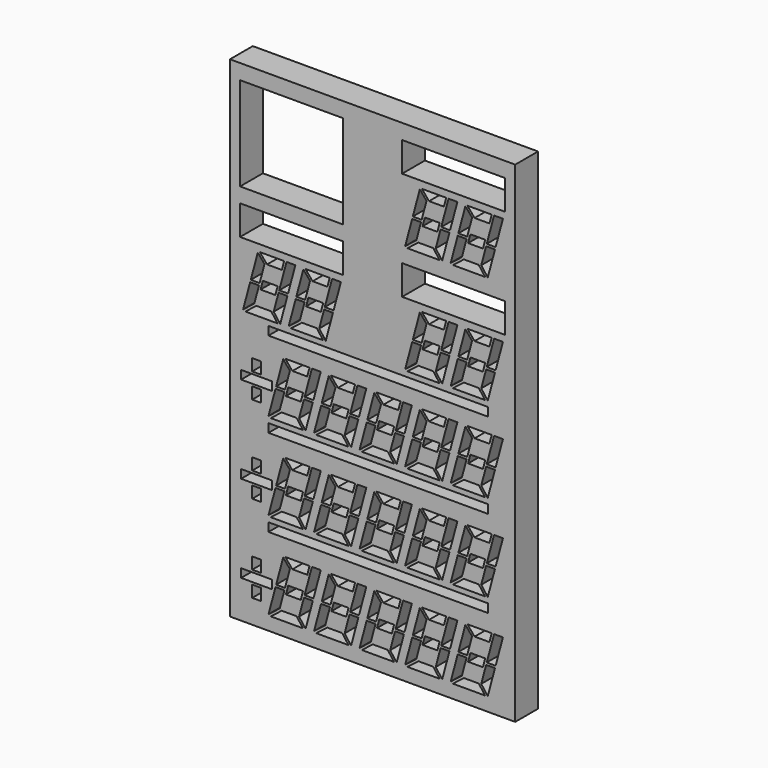
from build123d import *

# Parameters (mm, degrees)
F0_W     = 63.5
F0_H     = 109.22
F1_DEPTH = 6.35
F2_W     = 48.8092640617
F2_H     = 1.905
F2_W_2   = 1.905
F2_H_2   = 2.6035
F2_W_3   = 22.86
F2_H_3   = 6.604
F2_H_4   = 20.828
F3_DEPTH = 6.351


# Not quite as in the source:
# - a feature of the source that left no trace in its solid (it failed there, or was rolled back) is left out


with BuildPart() as f1:
    # F0 (on Front) → F1 (new body)
    with BuildSketch(Plane.XZ):
        Rectangle(F0_W, F0_H)
    extrude(amount=F1_DEPTH)

    # F2 (on face) → F3 (cut, through all)
    with BuildSketch(Plane.XZ.offset(6.35)):
        Polygon((26.5213785767, -38.9255), (21.1104505677, -38.9255), (22.7089353651, -40.8305), (26.0109353651, -40.8305), align=None)
        Polygon((29.0195, -38.9255), (27.0472988763, -38.9255), (25.4138805993, -45.0215), (27.3860817229, -45.0215), align=None)
        Polygon((27.2499635332, -45.5295), (25.2777624095, -45.5295), (24.1836844814, -49.6126544151), (25.6385600829, -51.5433395481), align=None)
        Polygon((22.1498008505, -40.9544571376), (20.6549496749, -39.1729628786), (19.0878388763, -45.0215), (21.06004, -45.0215), align=None)
        Polygon((17.888578235, -51.6255), (25.0643875098, -51.6255), (23.6288670444, -49.7205), (20.3268670444, -49.7205), align=None)
        Polygon((19.8801693423, -49.4248372408), (20.9239218102, -45.5295), (18.9517206865, -45.5295), (17.3857808211, -51.3736671393), align=None)
        Polygon((25.0751228105, -44.323), (21.7731228105, -44.323), (21.2626795989, -46.228), (24.5646795989, -46.228), align=None)
        Polygon((21.7731228105, -24.892), (21.2626795989, -26.797), (24.5646795989, -26.797), (25.0751228105, -24.892), align=None)
        Polygon((20.9239218102, -26.0985), (18.9517206865, -26.0985), (17.3857808211, -31.9426671393), (19.8801693423, -29.9938372408), align=None)
        Polygon((21.06004, -25.5905), (22.1498008505, -21.5234571376), (20.6549496749, -19.7419628786), (19.0878388763, -25.5905), align=None)
        Polygon((27.3860817229, -25.5905), (29.0195, -19.4945), (27.0472988763, -19.4945), (25.4138805993, -25.5905), align=None)
        Polygon((22.7089353651, -21.3995), (26.0109353651, -21.3995), (26.5213785767, -19.4945), (21.1104505677, -19.4945), align=None)
        Polygon((17.888578235, -32.1945), (25.0643875098, -32.1945), (23.6288670444, -30.2895), (20.3268670444, -30.2895), align=None)
        Polygon((27.2499635332, -26.0985), (25.2777624095, -26.0985), (24.1836844814, -30.1816544151), (25.6385600829, -32.1123395481), align=None)
        Polygon((21.7731228105, -5.461), (21.2626795989, -7.366), (24.5646795989, -7.366), (25.0751228105, -5.461), align=None)
        Polygon((20.9239218102, -6.6675), (18.9517206865, -6.6675), (17.3857808211, -12.5116671393), (19.8801693423, -10.5628372408), align=None)
        Polygon((21.06004, -6.1595), (22.1498008505, -2.0924571376), (20.6549496749, -0.3109628786), (19.0878388763, -6.1595), align=None)
        Polygon((27.3860817229, -6.1595), (29.0195, -0.0635), (27.0472988763, -0.0635), (25.4138805993, -6.1595), align=None)
        Polygon((22.7089353651, -1.9685), (26.0109353651, -1.9685), (26.5213785767, -0.0635), (21.1104505677, -0.0635), align=None)
        Polygon((17.888578235, -12.7635), (25.0643875098, -12.7635), (23.6288670444, -10.8585), (20.3268670444, -10.8585), align=None)
        Polygon((27.2499635332, -6.6675), (25.2777624095, -6.6675), (24.1836844814, -10.7506544151), (25.6385600829, -12.6813395481), align=None)
        Polygon((11.6340016105, -44.323), (11.1235583989, -46.228), (14.4255583989, -46.228), (14.9360016105, -44.323), align=None)
        Polygon((10.7848006102, -45.5295), (8.8125994865, -45.5295), (7.2466596211, -51.3736671393), (9.7410481423, -49.4248372408), align=None)
        Polygon((10.9209188, -45.0215), (12.0106796505, -40.9544571376), (10.5158284749, -39.1729628786), (8.9487176763, -45.0215), align=None)
        Polygon((17.2469605229, -45.0215), (18.8803788, -38.9255), (16.9081776763, -38.9255), (15.2747593993, -45.0215), align=None)
        Polygon((12.5698141651, -40.8305), (15.8718141651, -40.8305), (16.3822573767, -38.9255), (10.9713293677, -38.9255), align=None)
        Polygon((7.749457035, -51.6255), (14.9252663098, -51.6255), (13.4897458444, -49.7205), (10.1877458444, -49.7205), align=None)
        Polygon((17.1108423332, -45.5295), (15.1386412095, -45.5295), (14.0445632814, -49.6126544151), (15.4994388829, -51.5433395481), align=None)
        Polygon((11.6340016105, -24.892), (11.1235583989, -26.797), (14.4255583989, -26.797), (14.9360016105, -24.892), align=None)
        Polygon((10.7848006102, -26.0985), (8.8125994865, -26.0985), (7.2466596211, -31.9426671393), (9.7410481423, -29.9938372408), align=None)
        Polygon((10.9209188, -25.5905), (12.0106796505, -21.5234571376), (10.5158284749, -19.7419628786), (8.9487176763, -25.5905), align=None)
        Polygon((17.2469605229, -25.5905), (18.8803788, -19.4945), (16.9081776763, -19.4945), (15.2747593993, -25.5905), align=None)
        Polygon((12.5698141651, -21.3995), (15.8718141651, -21.3995), (16.3822573767, -19.4945), (10.9713293677, -19.4945), align=None)
        Polygon((7.749457035, -32.1945), (14.9252663098, -32.1945), (13.4897458444, -30.2895), (10.1877458444, -30.2895), align=None)
        Polygon((17.1108423332, -26.0985), (15.1386412095, -26.0985), (14.0445632814, -30.1816544151), (15.4994388829, -32.1123395481), align=None)
        Polygon((11.6340016105, -5.461), (11.1235583989, -7.366), (14.4255583989, -7.366), (14.9360016105, -5.461), align=None)
        Polygon((10.7848006102, -6.6675), (8.8125994865, -6.6675), (7.2466596211, -12.5116671393), (9.7410481423, -10.5628372408), align=None)
        Polygon((10.9209188, -6.1595), (12.0106796505, -2.0924571376), (10.5158284749, -0.3109628786), (8.9487176763, -6.1595), align=None)
        Polygon((17.2469605229, -6.1595), (18.8803788, -0.0635), (16.9081776763, -0.0635), (15.2747593993, -6.1595), align=None)
        Polygon((12.5698141651, -1.9685), (15.8718141651, -1.9685), (16.3822573767, -0.0635), (10.9713293677, -0.0635), align=None)
        Polygon((7.749457035, -12.7635), (14.9252663098, -12.7635), (13.4897458444, -10.8585), (10.1877458444, -10.8585), align=None)
        Polygon((17.1108423332, -6.6675), (15.1386412095, -6.6675), (14.0445632814, -10.7506544151), (15.4994388829, -12.6813395481), align=None)
        Polygon((1.4948804105, -44.323), (0.9844371989, -46.228), (4.2864371989, -46.228), (4.7968804105, -44.323), align=None)
        Polygon((0.6456794102, -45.5295), (-1.3265217135, -45.5295), (-2.8924615789, -51.3736671393), (-0.3980730577, -49.4248372408), align=None)
        Polygon((0.7817976, -45.0215), (1.8715584505, -40.9544571376), (0.3767072749, -39.1729628786), (-1.1904035237, -45.0215), align=None)
        Polygon((7.1078393229, -45.0215), (8.7412576, -38.9255), (6.7690564763, -38.9255), (5.1356381993, -45.0215), align=None)
        Polygon((2.4306929651, -40.8305), (5.7326929651, -40.8305), (6.2431361767, -38.9255), (0.8322081677, -38.9255), align=None)
        Polygon((-2.389664165, -51.6255), (4.7861451098, -51.6255), (3.3506246444, -49.7205), (0.0486246444, -49.7205), align=None)
        Polygon((6.9717211332, -45.5295), (4.9995200095, -45.5295), (3.9054420814, -49.6126544151), (5.3603176829, -51.5433395481), align=None)
        Polygon((1.4948804105, -24.892), (0.9844371989, -26.797), (4.2864371989, -26.797), (4.7968804105, -24.892), align=None)
        Polygon((0.6456794102, -26.0985), (-1.3265217135, -26.0985), (-2.8924615789, -31.9426671393), (-0.3980730577, -29.9938372408), align=None)
        Polygon((0.7817976, -25.5905), (1.8715584505, -21.5234571376), (0.3767072749, -19.7419628786), (-1.1904035237, -25.5905), align=None)
        Polygon((7.1078393229, -25.5905), (8.7412576, -19.4945), (6.7690564763, -19.4945), (5.1356381993, -25.5905), align=None)
        Polygon((2.4306929651, -21.3995), (5.7326929651, -21.3995), (6.2431361767, -19.4945), (0.8322081677, -19.4945), align=None)
        Polygon((-2.389664165, -32.1945), (4.7861451098, -32.1945), (3.3506246444, -30.2895), (0.0486246444, -30.2895), align=None)
        Polygon((6.9717211332, -26.0985), (4.9995200095, -26.0985), (3.9054420814, -30.1816544151), (5.3603176829, -32.1123395481), align=None)
        Polygon((1.4948804105, -5.461), (0.9844371989, -7.366), (4.2864371989, -7.366), (4.7968804105, -5.461), align=None)
        Polygon((0.6456794102, -6.6675), (-1.3265217135, -6.6675), (-2.8924615789, -12.5116671393), (-0.3980730577, -10.5628372408), align=None)
        Polygon((0.7817976, -6.1595), (1.8715584505, -2.0924571376), (0.3767072749, -0.3109628786), (-1.1904035237, -6.1595), align=None)
        Polygon((7.1078393229, -6.1595), (8.7412576, -0.0635), (6.7690564763, -0.0635), (5.1356381993, -6.1595), align=None)
        Polygon((2.4306929651, -1.9685), (5.7326929651, -1.9685), (6.2431361767, -0.0635), (0.8322081677, -0.0635), align=None)
        Polygon((-2.389664165, -12.7635), (4.7861451098, -12.7635), (3.3506246444, -10.8585), (0.0486246444, -10.8585), align=None)
        Polygon((6.9717211332, -6.6675), (4.9995200095, -6.6675), (3.9054420814, -10.7506544151), (5.3603176829, -12.6813395481), align=None)
        Polygon((-8.6442407895, -44.323), (-9.1546840011, -46.228), (-5.8526840011, -46.228), (-5.3422407895, -44.323), align=None)
        Polygon((-9.4934417898, -45.5295), (-11.4656429135, -45.5295), (-13.0315827789, -51.3736671393), (-10.5371942577, -49.4248372408), align=None)
        Polygon((-9.3573236, -45.0215), (-8.2675627495, -40.9544571376), (-9.7624139251, -39.1729628786), (-11.3295247237, -45.0215), align=None)
        Polygon((-3.0312818771, -45.0215), (-1.3978636, -38.9255), (-3.3700647237, -38.9255), (-5.0034830007, -45.0215), align=None)
        Polygon((-7.7084282349, -40.8305), (-4.4064282349, -40.8305), (-3.8959850233, -38.9255), (-9.3069130323, -38.9255), align=None)
        Polygon((-12.528785365, -51.6255), (-5.3529760902, -51.6255), (-6.7884965556, -49.7205), (-10.0904965556, -49.7205), align=None)
        Polygon((-3.1674000668, -45.5295), (-5.1396011905, -45.5295), (-6.2336791186, -49.6126544151), (-4.7788035171, -51.5433395481), align=None)
        Polygon((-8.6442407895, -24.892), (-9.1546840011, -26.797), (-5.8526840011, -26.797), (-5.3422407895, -24.892), align=None)
        Polygon((-9.4934417898, -26.0985), (-11.4656429135, -26.0985), (-13.0315827789, -31.9426671393), (-10.5371942577, -29.9938372408), align=None)
        Polygon((-9.3573236, -25.5905), (-8.2675627495, -21.5234571376), (-9.7624139251, -19.7419628786), (-11.3295247237, -25.5905), align=None)
        Polygon((-3.0312818771, -25.5905), (-1.3978636, -19.4945), (-3.3700647237, -19.4945), (-5.0034830007, -25.5905), align=None)
        Polygon((-7.7084282349, -21.3995), (-4.4064282349, -21.3995), (-3.8959850233, -19.4945), (-9.3069130323, -19.4945), align=None)
        Polygon((-12.528785365, -32.1945), (-5.3529760902, -32.1945), (-6.7884965556, -30.2895), (-10.0904965556, -30.2895), align=None)
        Polygon((-3.1674000668, -26.0985), (-5.1396011905, -26.0985), (-6.2336791186, -30.1816544151), (-4.7788035171, -32.1123395481), align=None)
        Polygon((-8.6442407895, -5.461), (-9.1546840011, -7.366), (-5.8526840011, -7.366), (-5.3422407895, -5.461), align=None)
        Polygon((-9.4934417898, -6.6675), (-11.4656429135, -6.6675), (-13.0315827789, -12.5116671393), (-10.5371942577, -10.5628372408), align=None)
        Polygon((-9.3573236, -6.1595), (-8.2675627495, -2.0924571376), (-9.7624139251, -0.3109628786), (-11.3295247237, -6.1595), align=None)
        Polygon((-3.0312818771, -6.1595), (-1.3978636, -0.0635), (-3.3700647237, -0.0635), (-5.0034830007, -6.1595), align=None)
        Polygon((-7.7084282349, -1.9685), (-4.4064282349, -1.9685), (-3.8959850233, -0.0635), (-9.3069130323, -0.0635), align=None)
        Polygon((-12.528785365, -12.7635), (-5.3529760902, -12.7635), (-6.7884965556, -10.8585), (-10.0904965556, -10.8585), align=None)
        Polygon((-3.1674000668, -6.6675), (-5.1396011905, -6.6675), (-6.2336791186, -10.7506544151), (-4.7788035171, -12.6813395481), align=None)
        Polygon((-19.0385835953, -45.2755), (-19.2938052011, -46.228), (-15.9918052011, -46.228), (-15.4813619895, -44.323), (-18.7833619895, -44.323), align=None)
        Polygon((-19.6325629898, -45.5295), (-21.6047641135, -45.5295), (-23.1707039789, -51.3736671393), (-20.6763154577, -49.4248372408), align=None)
        Polygon((-19.4964448, -45.0215), (-18.4066839495, -40.9544571376), (-19.9015351251, -39.1729628786), (-21.4686459237, -45.0215), align=None)
        Polygon((-13.1704030771, -45.0215), (-11.5369848, -38.9255), (-13.5091859237, -38.9255), (-15.1426042007, -45.0215), align=None)
        Polygon((-17.8475494349, -40.8305), (-14.5455494349, -40.8305), (-14.0351062233, -38.9255), (-19.4460342323, -38.9255), align=None)
        Polygon((-22.667906565, -51.6255), (-15.4920972902, -51.6255), (-16.9276177556, -49.7205), (-20.2296177556, -49.7205), align=None)
        Polygon((-13.3065212668, -45.5295), (-15.2787223905, -45.5295), (-16.3728003186, -49.6126544151), (-14.9179247171, -51.5433395481), align=None)
        Polygon((-18.7833619895, -24.892), (-19.2938052011, -26.797), (-15.9918052011, -26.797), (-15.4813619895, -24.892), align=None)
        Polygon((-19.6325629898, -26.0985), (-21.6047641135, -26.0985), (-23.1707039789, -31.9426671393), (-20.6763154577, -29.9938372408), align=None)
        Polygon((-19.4964448, -25.5905), (-18.4066839495, -21.5234571376), (-19.9015351251, -19.7419628786), (-21.4686459237, -25.5905), align=None)
        Polygon((-13.1704030771, -25.5905), (-11.5369848, -19.4945), (-13.5091859237, -19.4945), (-15.1426042007, -25.5905), align=None)
        Polygon((-17.8475494349, -21.3995), (-14.5455494349, -21.3995), (-14.0351062233, -19.4945), (-19.4460342323, -19.4945), align=None)
        Polygon((-22.667906565, -32.1945), (-15.4920972902, -32.1945), (-16.9276177556, -30.2895), (-20.2296177556, -30.2895), align=None)
        Polygon((-13.3065212668, -26.0985), (-15.2787223905, -26.0985), (-16.3728003186, -30.1816544151), (-14.9179247171, -32.1123395481), align=None)
        Polygon((-18.7833619895, -5.461), (-19.2938052011, -7.366), (-15.9918052011, -7.366), (-15.4813619895, -5.461), align=None)
        Polygon((-19.6325629898, -6.6675), (-21.6047641135, -6.6675), (-23.1707039789, -12.5116671393), (-20.6763154577, -10.5628372408), align=None)
        Polygon((-19.4964448, -6.1595), (-18.4066839495, -2.0924571376), (-19.9015351251, -0.3109628786), (-21.4686459237, -6.1595), align=None)
        Polygon((-13.1704030771, -6.1595), (-11.5369848, -0.0635), (-13.5091859237, -0.0635), (-15.1426042007, -6.1595), align=None)
        Polygon((-17.8475494349, -1.9685), (-14.5455494349, -1.9685), (-14.0351062233, -0.0635), (-19.4460342323, -0.0635), align=None)
        Polygon((-22.667906565, -12.7635), (-15.4920972902, -12.7635), (-16.9276177556, -10.8585), (-20.2296177556, -10.8585), align=None)
        Polygon((-13.3065212668, -6.6675), (-15.2787223905, -6.6675), (-16.3728003186, -10.7506544151), (-14.9179247171, -12.6813395481), align=None)
        Polygon((22.7089353651, 17.0815), (26.0109353651, 17.0815), (26.5213785767, 18.9865), (21.1104505677, 18.9865), align=None)
        Polygon((21.7731228105, 13.589), (21.2626795989, 11.684), (24.5646795989, 11.684), (25.0751228105, 13.589), align=None)
        Polygon((12.5698141651, 17.0815), (15.8718141651, 17.0815), (16.3822573767, 18.9865), (10.9713293677, 18.9865), align=None)
        Polygon((29.0195, 18.9865), (27.0472988763, 18.9865), (25.4138805993, 12.8905), (27.3860817229, 12.8905), align=None)
        Polygon((18.9517206865, 12.3825), (17.3857808211, 6.5383328607), (19.8801693423, 8.4871627592), (20.9239218102, 12.3825), align=None)
        Polygon((21.06004, 12.8905), (22.1498008505, 16.9575428624), (20.6549496749, 18.7390371214), (19.0878388763, 12.8905), align=None)
        Polygon((27.2499635332, 12.3825), (25.2777624095, 12.3825), (24.1836844814, 8.2993455849), (25.6385600829, 6.3686604519), align=None)
        Polygon((20.3268670444, 8.1915), (17.888578235, 6.2865), (25.0643875098, 6.2865), (23.6288670444, 8.1915), align=None)
        Polygon((15.4994388829, 6.3686604519), (17.1108423332, 12.3825), (15.1386412095, 12.3825), (14.0445632814, 8.2993455849), align=None)
        Polygon((18.8803788, 18.9865), (16.9081776763, 18.9865), (15.2747593993, 12.8905), (17.2469605229, 12.8905), align=None)
        Polygon((7.2466596211, 6.5383328607), (9.7410481423, 8.4871627592), (10.7848006102, 12.3825), (8.8125994865, 12.3825), align=None)
        Polygon((10.5158284749, 18.7390371214), (8.9487176763, 12.8905), (10.9209188, 12.8905), (12.0106796505, 16.9575428624), align=None)
        Polygon((14.9252663098, 6.2865), (13.4897458444, 8.1915), (10.1877458444, 8.1915), (7.749457035, 6.2865), align=None)
        Polygon((11.6340016105, 13.589), (11.1235583989, 11.684), (14.4255583989, 11.684), (14.9360016105, 13.589), align=None)
        Polygon((29.0195, 43.1165), (27.0472988763, 43.1165), (25.4138805993, 37.0205), (27.3860817229, 37.0205), align=None)
        Polygon((24.5646795989, 35.814), (25.0751228105, 37.719), (21.7731228105, 37.719), (21.2626795989, 35.814), align=None)
        Polygon((22.7089353651, 41.2115), (26.0109353651, 41.2115), (26.5213785767, 43.1165), (21.1104505677, 43.1165), align=None)
        Polygon((21.06004, 37.0205), (22.1498008505, 41.0875428624), (20.6549496749, 42.8690371214), (19.0878388763, 37.0205), align=None)
        Polygon((10.7848006102, 36.5125), (8.8125994865, 36.5125), (7.2466596211, 30.6683328607), (9.7410481423, 32.6171627592), align=None)
        Polygon((20.9239218102, 36.5125), (18.9517206865, 36.5125), (17.3857808211, 30.6683328607), (19.8801693423, 32.6171627592), align=None)
        Polygon((10.5158284749, 42.8690371214), (8.9487176763, 37.0205), (10.9209188, 37.0205), (12.0106796505, 41.0875428624), align=None)
        Polygon((27.2499635332, 36.5125), (25.2777624095, 36.5125), (24.1836844814, 32.4293455849), (25.6385600829, 30.4986604519), align=None)
        Polygon((15.4994388829, 30.4986604519), (17.1108423332, 36.5125), (15.1386412095, 36.5125), (14.0445632814, 32.4293455849), align=None)
        Polygon((17.2469605229, 37.0205), (18.8803788, 43.1165), (16.9081776763, 43.1165), (15.2747593993, 37.0205), align=None)
        Polygon((14.9252663098, 30.4165), (13.4897458444, 32.3215), (10.1877458444, 32.3215), (7.749457035, 30.4165), align=None)
        Polygon((16.3822573767, 43.1165), (10.9713293677, 43.1165), (12.5698141651, 41.2115), (15.8718141651, 41.2115), align=None)
        Polygon((17.888578235, 30.4165), (25.0643875098, 30.4165), (23.6288670444, 32.3215), (20.3268670444, 32.3215), align=None)
        Polygon((11.6340016105, 37.719), (11.1235583989, 35.814), (14.4255583989, 35.814), (14.9360016105, 37.719), align=None)
        Polygon((-10.4294399171, 6.3686604519), (-8.8180364668, 12.3825), (-10.7902375905, 12.3825), (-11.8843155186, 8.2993455849), align=None)
        Polygon((-18.8210394771, 12.8905), (-17.1876212, 18.9865), (-19.1598223237, 18.9865), (-20.7932406007, 12.8905), align=None)
        Polygon((-15.1440781898, 12.3825), (-17.1162793135, 12.3825), (-18.6822191789, 6.5383328607), (-16.1878306577, 8.4871627592), align=None)
        Polygon((-25.2831993898, 12.3825), (-27.2554005135, 12.3825), (-28.8213403789, 6.5383328607), (-26.3269518577, 8.4871627592), align=None)
        Polygon((-19.6857426233, 18.9865), (-25.0966706323, 18.9865), (-23.4981858349, 17.0815), (-20.1961858349, 17.0815), align=None)
        Polygon((-9.5466214233, 18.9865), (-14.9575494323, 18.9865), (-13.3590646349, 17.0815), (-10.0570646349, 17.0815), align=None)
        Polygon((-15.4130503251, 18.7390371214), (-16.9801611237, 12.8905), (-15.00796, 12.8905), (-13.9181991495, 16.9575428624), align=None)
        Polygon((-25.5521715251, 18.7390371214), (-27.1192823237, 12.8905), (-25.1470812, 12.8905), (-24.0573203495, 16.9575428624), align=None)
        Polygon((-28.318542965, 6.2865), (-21.1427336902, 6.2865), (-22.5782541556, 8.1915), (-25.8802541556, 8.1915), align=None)
        Polygon((-18.179421765, 6.2865), (-11.0036124902, 6.2865), (-12.4391329556, 8.1915), (-15.7411329556, 8.1915), align=None)
        Polygon((-8.6819182771, 12.8905), (-7.0485, 18.9865), (-9.0207011237, 18.9865), (-10.6541194007, 12.8905), align=None)
        Polygon((-20.5685611171, 6.3686604519), (-18.9571576668, 12.3825), (-20.9293587905, 12.3825), (-22.0234367186, 8.2993455849), align=None)
        Polygon((-14.2948771895, 13.589), (-14.8053204011, 11.684), (-11.5033204011, 11.684), (-10.9928771895, 13.589), align=None)
        Polygon((-24.4339983895, 13.589), (-24.9444416011, 11.684), (-21.6424416011, 11.684), (-21.1319983895, 13.589), align=None)
        with Locations((1.233928052, -34.29)):
            Rectangle(F2_W, F2_H)
        with Locations((1.233928052, -14.859)):
            Rectangle(F2_W, F2_H)
        Polygon((-25.8445, -44.323), (-29.2735, -44.323), (-29.2735, -46.228), (-22.4155, -46.228), (-22.4155, -45.2755), (-22.4155, -44.323), align=None)
        Polygon((-24.892, -41.2115), (-26.797, -41.2115), (-26.797, -43.815), (-25.8445, -43.815), (-24.892, -43.815), align=None)
        with Locations((-25.8445, -48.03775)):
            Rectangle(F2_W_2, F2_H_2)
        with Locations((1.233928052, 4.191)):
            Rectangle(F2_W, F2_H)
        with Locations((17.9978545693, 23.8125)):
            Rectangle(F2_W_3, F2_H_3)
        with Locations((17.9978545693, 47.9425)):
            Rectangle(F2_W_3, F2_H_3)
        with Locations((-18.0701454307, 23.8125)):
            Rectangle(F2_W_3, F2_H_3)
        with Locations((-18.0701454307, 40.8305)):
            Rectangle(F2_W_3, F2_H_4)
        Polygon((-22.4155, -24.892), (-25.8445, -24.892), (-29.2735, -24.892), (-29.2735, -26.797), (-22.4155, -26.797), (-22.4155, -25.8445), align=None)
        Polygon((-24.892, -21.7805), (-26.797, -21.7805), (-26.797, -24.384), (-25.8445, -24.384), (-24.892, -24.384), align=None)
        with Locations((-25.8445, -28.60675)):
            Rectangle(F2_W_2, F2_H_2)
        Polygon((-22.4155, -5.461), (-25.8445, -5.461), (-29.2735, -5.461), (-29.2735, -7.366), (-22.4155, -7.366), (-22.4155, -6.4135), align=None)
        Polygon((-24.892, -2.3495), (-26.797, -2.3495), (-26.797, -4.953), (-25.8445, -4.953), (-24.892, -4.953), align=None)
        with Locations((-25.8445, -9.17575)):
            Rectangle(F2_W_2, F2_H_2)
    extrude(amount=-F3_DEPTH, mode=Mode.SUBTRACT)


solid = f1.part
